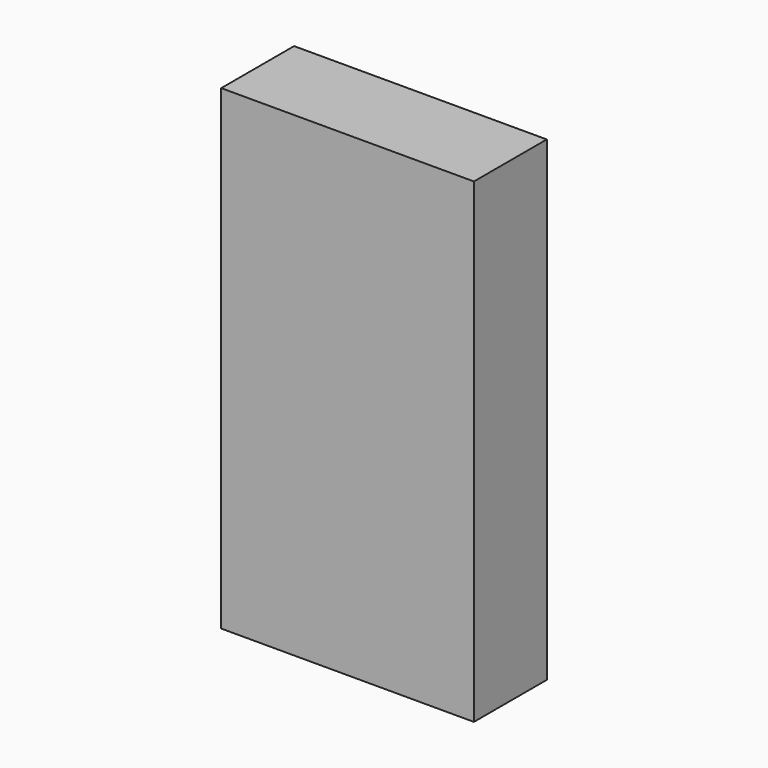
from build123d import *

# Parameters (mm, degrees)
F0_W     = 52.8712859377
F0_H     = 99.5555073023
F1_DEPTH = 19.05


# Not quite as in the source:
# - a length typed as a fraction of an inch, garbled in the dataset ("3 / 203.2 mm" for 3/8 in), is restored


with BuildPart() as f1:
    # F0 (on Front) → F1 (new body)
    with BuildSketch(Plane.XZ):
        with Locations((-37.12239163, 4.9215294421)):
            Rectangle(F0_W, F0_H)
    extrude(amount=F1_DEPTH)


solid = f1.part
